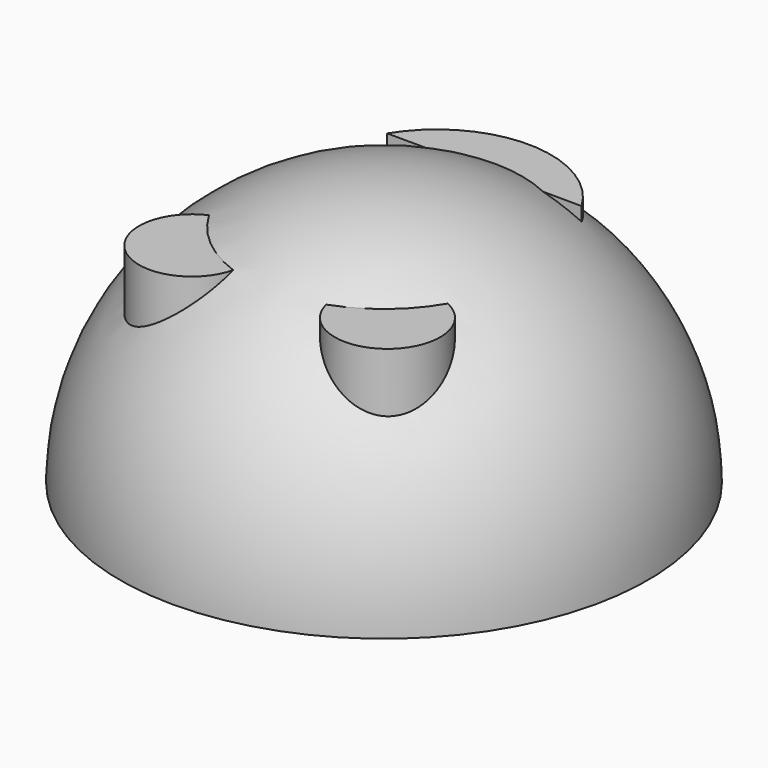
from build123d import *

# Parameters (mm, degrees)
F1_ANGLE = 180
F2_R     = 2.54
F4_DEPTH = 10.8204


with BuildPart() as f1:
    # F0 (on Top) → F1 (revolve)
    with BuildSketch(Plane.XY):
        with BuildLine():
            Line((0, 0), (0, 12.7))
            ThreePointArc((0, 12.7), (-12.7, 0), (0, -12.7))
            Line((0, -12.7), (0, 0))
        make_face()
    revolve(axis=Axis((0, 0, 0), (0, 1, 0)), revolution_arc=F1_ANGLE)

    # F3 (on Top) + F2 (on Top) → F4 (join)
    with BuildSketch(Plane.XY):
        with BuildLine():
            Line((-4.6839732677, 6.046992261), (4.7185341828, 5.9900078923))
            ThreePointArc((4.7185341828, 5.9900078923), (0.0333416464, 8.6686206572), (-4.6839732677, 6.046992261))
        make_face()
    with BuildSketch(Plane.XY):
        with Locations((4.695169162, -5.6601171382)):
            Circle(F2_R)
        with Locations((-4.7209146433, -5.6601171382)):
            Circle(F2_R)
    extrude(amount=F4_DEPTH)


solid = f1.part
